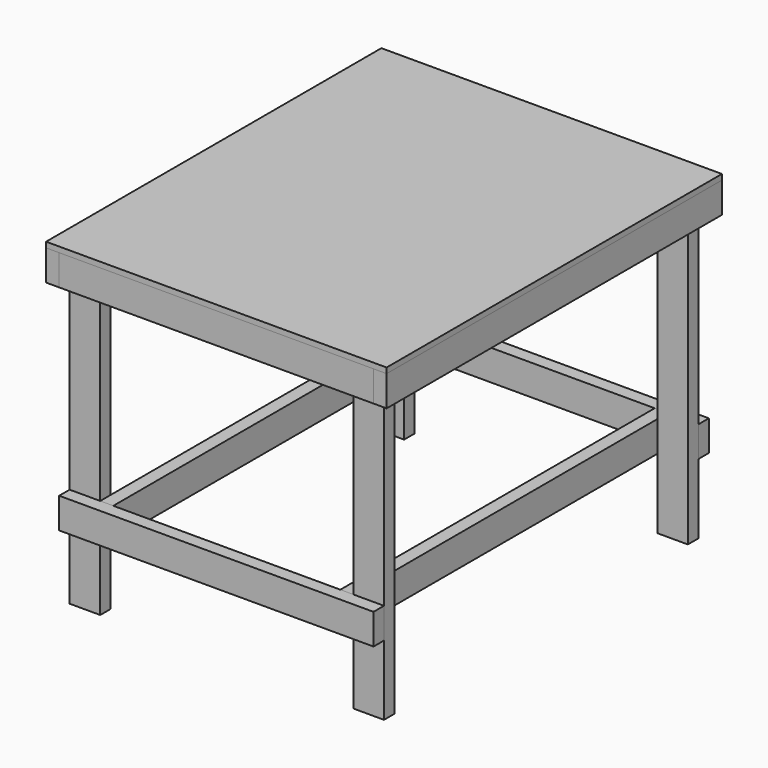
from build123d import *

# Parameters (mm, degrees)
F6_W          = 88.9
F6_H          = 38.1
F7_DEPTH      = 711.2
F7_DEPTH_BACK = 203.2
F8_DEPTH      = 88.9
F9_DEPTH      = 88.9
F11_W         = 1181.1
F11_H         = 88.9
F11_W_2       = 38.1
F12_DEPTH     = 38.1
F14_W         = 952.5
F14_H         = 1219.2
F14_W_2       = 38.1
F15_DEPTH     = 15.875


# Not quite as in the source:
# - a length typed as a fraction of an inch, garbled in the dataset ("3 / 203.2 mm" for 3/8 in), is restored


with BuildPart() as f7:
    # F6 (on Top) → F7 (new body, two sides)
    with BuildSketch(Plane.XY) as f7_sk:
        with Locations((412.75, -552.45)):
            Rectangle(F6_W, F6_H)
    extrude(amount=F7_DEPTH)
    extrude(f7_sk.sketch, amount=-F7_DEPTH_BACK)


with BuildPart() as f7b:
    # F6 (on Top) → F7, piece 2 (new body, two sides)
    with BuildSketch(Plane.XY) as f7_2_sk:
        with Locations((412.75, 552.45)):
            Rectangle(F6_W, F6_H)
    extrude(amount=F7_DEPTH)
    extrude(f7_2_sk.sketch, amount=-F7_DEPTH_BACK)


with BuildPart() as f7c:
    # F6 (on Top) → F7, piece 3 (new body, two sides)
    with BuildSketch(Plane.XY) as f7_3_sk:
        with Locations((-412.75, 552.45)):
            Rectangle(F6_W, F6_H)
    extrude(amount=F7_DEPTH)
    extrude(f7_3_sk.sketch, amount=-F7_DEPTH_BACK)


with BuildPart() as f7d:
    # F6 (on Top) → F7, piece 4 (new body, two sides)
    with BuildSketch(Plane.XY) as f7_4_sk:
        with Locations((-412.75, -552.45)):
            Rectangle(F6_W, F6_H)
    extrude(amount=F7_DEPTH)
    extrude(f7_4_sk.sketch, amount=-F7_DEPTH_BACK)


with BuildPart() as f8:
    # F6 (on Top) → F8 (new body)
    with BuildSketch(Plane.XY):
        Polygon((-330.2, 571.5), (330.2, 571.5), (368.3, 571.5), (457.2, 571.5), (457.2, 609.6), (-457.2, 609.6), (-457.2, 571.5), (-368.3, 571.5), align=None)
    extrude(amount=F8_DEPTH)


with BuildPart() as f8b:
    # F6 (on Top) → F8, piece 2 (new body)
    with BuildSketch(Plane.XY):
        Polygon((368.3, -571.5), (330.2, -571.5), (-330.2, -571.5), (-368.3, -571.5), (-457.2, -571.5), (-457.2, -609.6), (457.2, -609.6), (457.2, -571.5), align=None)
    extrude(amount=F8_DEPTH)


with BuildPart() as f9:
    # F6 (on Top) → F9 (new body)
    with BuildSketch(Plane.XY):
        Polygon((-330.2, -571.5), (-330.2, 571.5), (-368.3, 571.5), (-368.3, 533.4), (-368.3, -533.4), (-368.3, -571.5), align=None)
    extrude(amount=F9_DEPTH)


with BuildPart() as f9b:
    # F6 (on Top) → F9, piece 2 (new body)
    with BuildSketch(Plane.XY):
        Polygon((368.3, 571.5), (330.2, 571.5), (330.2, -571.5), (368.3, -571.5), (368.3, -533.4), (368.3, 533.4), align=None)
    extrude(amount=F9_DEPTH)


with BuildPart() as f10_1:
    # F10: copy of F8
    add(f8.part.moved(Location((0, 0, 622.3))))


with BuildPart() as f10_2:
    # F10: copy of F8b
    add(f8b.part.moved(Location((0, 0, 622.3))))


with BuildPart() as f12:
    # F11 (on face) → F12 (new body)
    with BuildSketch(Plane.YZ.offset(457.2)):
        with Locations((19.05, 666.75)):
            Rectangle(F11_W, F11_H)
        with Locations((-590.55, 666.75)):
            Rectangle(F11_W_2, F11_H)
    extrude(amount=F12_DEPTH)


with BuildPart() as f13_1:
    # F13: copy of F12
    add(f12.part.moved(Location((-952.5, 0, 0))))


with BuildPart() as f15:
    # F14 (on face) → F15 (new body)
    with BuildSketch(Plane.XY.offset(711.2)):
        with Locations((-19.05, 0)):
            Rectangle(F14_W, F14_H)
        with Locations((476.25, 0)):
            Rectangle(F14_W_2, F14_H)
    extrude(amount=F15_DEPTH)


solid = Compound([f7.part, f7b.part, f7c.part, f7d.part, f8.part, f8b.part, f9.part, f9b.part, f10_1.part, f10_2.part, f12.part, f13_1.part, f15.part])
